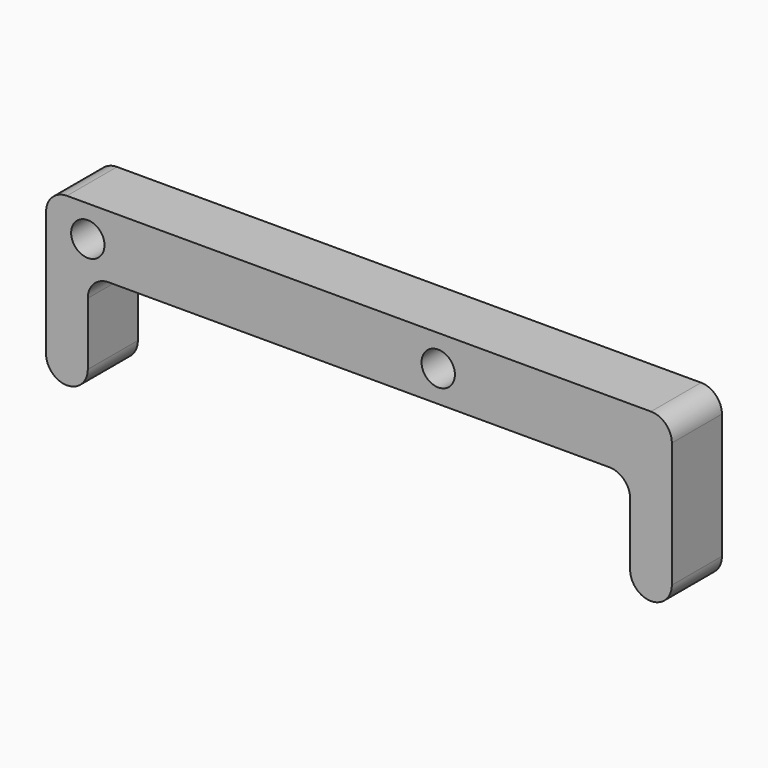
from build123d import *

# Parameters (mm, degrees)
F0_R     = 4
F0_W     = 10
F0_H     = 25
F1_DEPTH = 15
F2_R     = 4.99999


# Not quite as in the source:
# - a fillet or chamfer is up to 0.001 mm smaller than in the source, because OpenCascade refuses the exact size


with BuildPart() as f1:
    # F0 (on Front) → F1 (new body)
    with BuildSketch(Plane.XZ):
        Polygon((56, 7.5), (-94, 7.5), (-94, -7.5), (-84, -7.5), (46, -7.5), (56, -7.5), align=None)
        with Locations((-84, 0)):
            Circle(F0_R, mode=Mode.SUBTRACT)
        Circle(F0_R, mode=Mode.SUBTRACT)
        with Locations((-89, -20)):
            Rectangle(F0_W, F0_H)
        with Locations((51, -20)):
            Rectangle(F0_W, F0_H)
    extrude(amount=F1_DEPTH)

    # F2 (radius 5 in the source; OpenCascade refuses exactly that, so slightly less here)
    f2_edges = [f1.edges().sort_by_distance(p)[0] for p in [
        (-84, -7.5, -7.5),
        (46, -7.5, -7.5),
        (56, -7.5, 7.5),
        (56, -7.5, -32.5),
        (46, -7.5, -32.5),
        (-94, -7.5, -32.5),
        (-84, -7.5, -32.5),
        (-94, -7.5, 7.5),
    ]]
    fillet(f2_edges, radius=F2_R)


solid = f1.part
